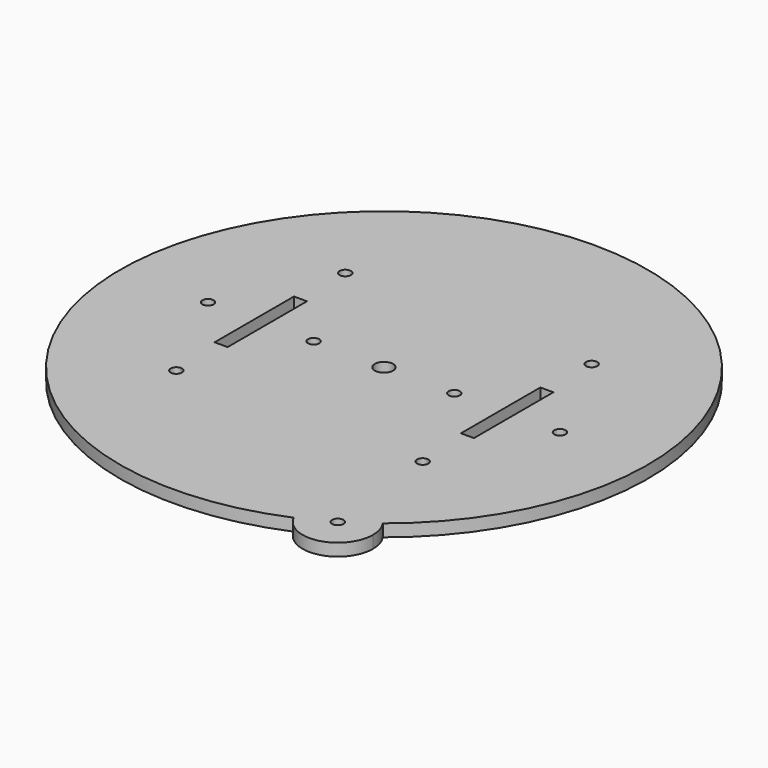
from build123d import *

# Parameters (mm, degrees)
F0_R     = 75
F1_DEPTH = 3.5
F2_R     = 1.6
F3_DEPTH = 3.5
F5_DEPTH = 3.5
F6_R     = 1.6
F7_DEPTH = 3.5
F8_W     = 1.85
F8_H     = 28.2
F9_DEPTH = 3.501


with BuildPart() as f1:
    # F0 (on Top) → F1 (new body)
    with BuildSketch(Plane.XY):
        Circle(F0_R)
    extrude(amount=F1_DEPTH)

    # F2 (on Top) → F3 (cut)
    with BuildSketch(Plane.XY):
        with BuildLine():
            ThreePointArc((-35, -28.4), (-36.1313708499, -31.1313708499), (-33.4, -30))
            Line((-33.4, -30), (-35, -30))
            Line((-35, -30), (-35, -28.4))
        make_face()
        with BuildLine():
            Line((-35, -30), (-33.4, -30))
            ThreePointArc((-33.4, -30), (-33.8686291501, -28.8686291501), (-35, -28.4))
            Line((-35, -28.4), (-35, -30))
        make_face()
        with Locations((-50, 0)):
            Circle(F2_R)
        with BuildLine():
            ThreePointArc((51.6, 0), (50, 1.6), (48.4, 0))
            ThreePointArc((48.4, 0), (50, -1.6), (51.6, 0))
        make_face()
        with BuildLine():
            ThreePointArc((35, -28.4), (33.8686291501, -28.8686291501), (33.4, -30))
            Line((33.4, -30), (35, -30))
            Line((35, -30), (35, -28.4))
        make_face()
        with BuildLine():
            Line((35, -30), (33.4, -30))
            ThreePointArc((33.4, -30), (35, -31.6), (36.6, -30))
            ThreePointArc((36.6, -30), (36.1313708499, -28.8686291501), (35, -28.4))
            Line((35, -28.4), (35, -30))
        make_face()
        with BuildLine():
            ThreePointArc((-33.4, 30), (-36.1313708499, 31.1313708499), (-35, 28.4))
            Line((-35, 28.4), (-35, 30))
            Line((-35, 30), (-33.4, 30))
        make_face()
        with BuildLine():
            Line((-35, 30), (-35, 28.4))
            ThreePointArc((-35, 28.4), (-33.8686291501, 28.8686291501), (-33.4, 30))
            Line((-33.4, 30), (-35, 30))
        make_face()
        with BuildLine():
            ThreePointArc((-18.4, 0), (-20, 1.6), (-21.6, 0))
            Line((-21.6, 0), (-20, 0))
            Line((-20, 0), (-18.4, 0))
        make_face()
        with BuildLine():
            Line((-20, 0), (-21.6, 0))
            ThreePointArc((-21.6, 0), (-20, -1.6), (-18.4, 0))
            Line((-18.4, 0), (-20, 0))
        make_face()
        with BuildLine():
            ThreePointArc((33.4, 30), (33.8686291501, 28.8686291501), (35, 28.4))
            Line((35, 28.4), (35, 30))
            Line((35, 30), (33.4, 30))
        make_face()
        with BuildLine():
            Line((35, 30), (35, 28.4))
            ThreePointArc((35, 28.4), (36.1313708499, 28.8686291501), (36.6, 30))
            ThreePointArc((36.6, 30), (35, 31.6), (33.4, 30))
            Line((33.4, 30), (35, 30))
        make_face()
        with BuildLine():
            ThreePointArc((18.4, 0), (20, -1.6), (21.6, 0))
            Line((21.6, 0), (20, 0))
            Line((20, 0), (18.4, 0))
        make_face()
        with BuildLine():
            Line((20, 0), (21.6, 0))
            ThreePointArc((21.6, 0), (20, 1.6), (18.4, 0))
            Line((18.4, 0), (20, 0))
        make_face()
        with BuildLine():
            ThreePointArc((2.6, 0), (0, 2.6), (-2.6, 0))
            Line((-2.6, 0), (2.6, 0))
        make_face()
        with BuildLine():
            Line((2.6, 0), (-2.6, 0))
            ThreePointArc((-2.6, 0), (0, -2.6), (2.6, 0))
        make_face()
    extrude(amount=F3_DEPTH, mode=Mode.SUBTRACT)

    # F4 (on face) → F5 (join)
    with BuildSketch(Plane.XY.offset(3.5)):
        with BuildLine():
            ThreePointArc((29.5025076199, -68.9536224149), (40.7469515469, -74.139754822), (48.4136259754, -64.4157848623))
            ThreePointArc((48.4136259754, -64.4157848623), (47.9604080116, -61.4393855689), (46.6418354247, -58.732777801))
            ThreePointArc((46.6418354247, -58.732777801), (38.4136259754, -64.4157848623), (29.5025076199, -68.9536224149))
        make_face()
    extrude(amount=-F5_DEPTH)

    # F6 (on face) → F7 (cut)
    with BuildSketch(Plane.XY.offset(3.5)):
        with Locations((38.4136259754, -64.4157848623)):
            Circle(F6_R)
    extrude(amount=-F7_DEPTH, mode=Mode.SUBTRACT)

    # F8 (on face) → F9 (cut, through all)
    with BuildSketch(Plane.XY.offset(3.5)):
        with Locations((-34.075, 0)):
            Rectangle(F8_W, F8_H)
        with Locations((-35.925, 0)):
            Rectangle(F8_W, F8_H)
        with Locations((35.925, 0)):
            Rectangle(F8_W, F8_H)
        with Locations((34.075, 0)):
            Rectangle(F8_W, F8_H)
    extrude(amount=-F9_DEPTH, mode=Mode.SUBTRACT)


solid = f1.part
